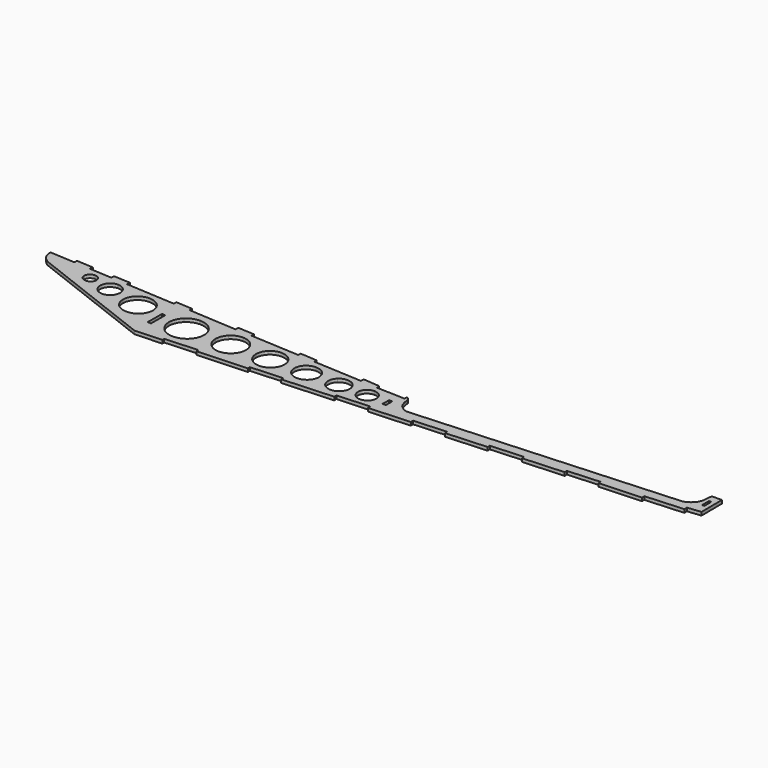
from build123d import *

# Parameters (mm, degrees)
F1_DEPTH = 3


# Not quite as in the source:
# - ends of sketch curves that miss each other by under 0.0002 mm in the source are joined
# - the dataset's text gives a spline's control points without its knots; the knots are read off the source's solid


with BuildPart() as f1:
    # F0 (on Top) → F1 (new body)
    with BuildSketch(Plane.XY):
        with BuildLine():
            Line((-283.705754, 26.242544), (-306.531989, 27.597216))
            Line((-306.531989, 27.597216), (-306.532132, 27.597217))
            add(Edge.make_bspline(
                [(-299.741399, 15.362947), (-303.248377, 18.203654), (-306.376642, 20.600294), (-306.532132, 27.597217)],
                knots=[0, 0, 0, 0, 1, 1, 1, 1], degree=3))
            Line((-299.741399, 15.362947), (-184.519619, -29.245478))
            Line((-184.519619, -29.245478), (-159.730079, -28.231688))
            Line((-159.730079, -28.231688), (-159.826994, -26.085226))
            Line((-159.826994, -26.085226), (-130.061797, -24.367861))
            Line((-130.061797, -24.367861), (-129.836804, -26.557253))
            Line((-129.836804, -26.557253), (-84.689902, -24.352981))
            Line((-84.689902, -24.352981), (-84.767699, -22.055153))
            Line((-84.767699, -22.055153), (-55.548697, -20.399041))
            Line((-55.548697, -20.399041), (-55.548607, -22.720141))
            Line((-55.548607, -22.720141), (-9.183299, -20.091946))
            Line((-9.183299, -20.091946), (-9.271814, -17.503366))
            Line((-9.271814, -17.503366), (20.343608, -15.913178))
            Line((20.343608, -15.913178), (20.340608, -18.583546))
            Line((20.340608, -18.583546), (57.798675, -16.459291))
            Line((57.798675, -16.459291), (57.7464, -13.835738))
            Line((57.7464, -13.835738), (87.580411, -12.096743))
            Line((87.580411, -12.096743), (87.59016, -14.588986))
            Line((87.59016, -14.588986), (124.670723, -12.419453))
            Line((124.670723, -12.419453), (124.718948, -9.896806))
            Line((124.718948, -9.896806), (154.696283, -8.076346))
            Line((154.696283, -8.076346), (154.845886, -10.628431))
            Line((154.845886, -10.628431), (191.943908, -8.450521))
            Line((191.943908, -8.450521), (191.926133, -5.905456))
            Line((191.926133, -5.905456), (221.443763, -4.073589))
            Line((221.443763, -4.073589), (221.435063, -6.558054))
            Line((221.435063, -6.558054), (259.473166, -4.558058))
            Line((259.473166, -4.558058), (259.447741, -1.913701))
            Line((259.447741, -1.913701), (294.319246, 0.265919))
            Line((294.319246, 0.265919), (294.223268, 3.278107))
            Line((294.223268, 3.278107), (306.532133, 4.590359))
            Line((306.532133, 4.590359), (306.343778, 28.117319))
            Line((306.343778, 28.117319), (298.342261, 27.997296))
            add(Edge.make_bspline(
                [(296.993228, 26.853134), (296.9935997444, 26.8539578555), (296.9936022923, 26.8539764219), (297.0233010775, 26.9195878034), (297.59233225, 28.1424128125), (298.342261, 27.997296)],
                knots=[0, 0, 0, 0, 0.0208333333, 0.03125, 1, 1, 1, 1], degree=3))
            Line((296.993228, 26.853134), (296.221861, 19.115617))
            add(Edge.make_bspline(
                [(285.733358, 8.770229), (290.415421, 10.119847), (295.053645, 13.441656), (296.221861, 19.115617)],
                knots=[0, 0, 0, 0, 1, 1, 1, 1], degree=3))
            Line((285.733358, 8.770229), (45.614513, -5.689073))
            add(Edge.make_bspline(
                [(38.011028, -1.579014), (40.407038, -3.364501), (42.648293, -5.614231), (45.614513, -5.689073)],
                knots=[0, 0, 0, 0, 1, 1, 1, 1], degree=3))
            add(Edge.make_bspline(
                [(34.690373, 8.210849), (35.274518, 4.947562), (35.678985, 1.684274), (38.011028, -1.579014)],
                knots=[0, 0, 0, 0, 1, 1, 1, 1], degree=3))
            add(Edge.make_bspline(
                [(31.92624, 11.727944), (33.14685, 10.854816), (34.877056, 10.491269), (34.690373, 8.210849)],
                knots=[0, 0, 0, 0, 1, 1, 1, 1], degree=3))
            Line((31.92624, 11.727944), (31.563826, 8.894204))
            Line((31.563826, 8.894204), (5.671996, 9.872969))
            Line((5.671996, 9.872969), (5.442765, 12.755872))
            Line((5.442765, 12.755872), (-9.382657, 14.013689))
            Line((-9.382657, 14.013689), (-9.615119, 10.891514))
            Line((-9.615119, 10.891514), (-53.849827, 13.259099))
            Line((-53.849827, 13.259099), (-54.080699, 15.881864))
            Line((-54.080699, 15.881864), (-69.487109, 16.950734))
            Line((-69.487109, 16.950734), (-69.592109, 14.198721))
            Line((-69.592109, 14.198721), (-114.174487, 16.652534))
            Line((-114.174487, 16.652534), (-114.050662, 19.463377))
            Line((-114.050662, 19.463377), (-129.098009, 20.234429))
            Line((-129.098009, 20.234429), (-129.237682, 17.136239))
            Line((-129.237682, 17.136239), (-173.38947, 19.880084))
            Line((-173.38947, 19.880084), (-173.40882, 22.677831))
            Line((-173.40882, 22.677831), (-188.406352, 23.557964))
            Line((-188.406352, 23.557964), (-188.417602, 20.663534))
            Line((-188.417602, 20.663534), (-233.27778, 23.322291))
            Line((-233.27778, 23.322291), (-233.11896, 26.423699))
            Line((-233.11896, 26.423699), (-248.233484, 27.111472))
            Line((-248.233484, 27.111472), (-248.199509, 24.138562))
            Line((-248.199509, 24.138562), (-268.624522, 25.372394))
            Line((-268.624522, 25.372394), (-268.486409, 28.327589))
            Line((-268.486409, 28.327589), (-283.648755, 29.245477))
            Line((-283.648755, 29.245477), (-283.705754, 26.242544))
        make_face()
        Polygon((-185.149065, -13.210493), (-184.989022, 2.952562), (-181.948447, 2.952562), (-181.948447, -13.370521), align=None, mode=Mode.SUBTRACT)
        with BuildLine():
            add(Edge.make_bspline(
                [(-157.220309, 11.895809), (-148.361018, 11.895807), (-141.179144, 4.900395), (-141.179144, -3.728881)],
                knots=[0, 0, 0, 0, 1, 1, 1, 1], degree=3))
            add(Edge.make_bspline(
                [(-141.179144, -3.728881), (-141.179142, -7.872807), (-142.869188, -11.847009), (-145.87749, -14.777209)],
                knots=[0, 0, 0, 0, 1, 1, 1, 1], degree=3))
            add(Edge.make_bspline(
                [(-145.87749, -14.777209), (-148.885792, -17.707408), (-152.965926, -19.353577), (-157.220309, -19.353578)],
                knots=[0, 0, 0, 0, 1, 1, 1, 1], degree=3))
            add(Edge.make_bspline(
                [(-157.220309, -19.353578), (-161.474694, -19.353579), (-165.55483, -17.707411), (-168.563134, -14.777211)],
                knots=[0, 0, 0, 0, 1, 1, 1, 1], degree=3))
            add(Edge.make_bspline(
                [(-168.563134, -14.777211), (-171.571438, -11.847012), (-173.261484, -7.872808), (-173.261482, -3.728881)],
                knots=[0, 0, 0, 0, 1, 1, 1, 1], degree=3))
            add(Edge.make_bspline(
                [(-173.261482, -3.728881), (-173.261482, 0.415045), (-171.571435, 4.389246), (-168.563131, 7.319444)],
                knots=[0, 0, 0, 0, 1, 1, 1, 1], degree=3))
            add(Edge.make_bspline(
                [(-168.563131, 7.319444), (-165.554828, 10.249642), (-161.474693, 11.89581), (-157.220309, 11.895809)],
                knots=[0, 0, 0, 0, 1, 1, 1, 1], degree=3))
        make_face(mode=Mode.SUBTRACT)
        with BuildLine():
            add(Edge.make_bspline(
                [(-107.474743, 6.629061), (-104.874921, 4.035491), (-103.414356, 0.517854), (-103.414357, -3.150008)],
                knots=[0, 0, 0, 0, 1, 1, 1, 1], degree=3))
            add(Edge.make_bspline(
                [(-103.414357, -3.150008), (-103.414359, -10.787934), (-109.621049, -16.979695), (-117.277387, -16.979694)],
                knots=[0, 0, 0, 0, 1, 1, 1, 1], degree=3))
            add(Edge.make_bspline(
                [(-117.277387, -16.979694), (-124.933725, -16.979695), (-131.140415, -10.787934), (-131.140417, -3.150008)],
                knots=[0, 0, 0, 0, 1, 1, 1, 1], degree=3))
            add(Edge.make_bspline(
                [(-131.140417, -3.150008), (-131.140418, 0.517854), (-129.679853, 4.035491), (-127.080031, 6.629061)],
                knots=[0, 0, 0, 0, 1, 1, 1, 1], degree=3))
            add(Edge.make_bspline(
                [(-127.080031, 6.629061), (-124.480208, 9.222632), (-120.954092, 10.679685), (-117.277387, 10.679684)],
                knots=[0, 0, 0, 0, 1, 1, 1, 1], degree=3))
            add(Edge.make_bspline(
                [(-117.277387, 10.679684), (-113.600682, 10.679685), (-110.074566, 9.222632), (-107.474743, 6.629061)],
                knots=[0, 0, 0, 0, 1, 1, 1, 1], degree=3))
        make_face(mode=Mode.SUBTRACT)
        with BuildLine():
            add(Edge.make_bspline(
                [(-71.752302, 5.620215), (-69.311057, 3.220874), (-67.939581, -0.033331), (-67.939582, -3.426511)],
                knots=[0, 0, 0, 0, 1, 1, 1, 1], degree=3))
            add(Edge.make_bspline(
                [(-67.939582, -3.426511), (-67.939585, -10.49244), (-73.767691, -16.220506), (-80.957025, -16.220506)],
                knots=[0, 0, 0, 0, 1, 1, 1, 1], degree=3))
            add(Edge.make_bspline(
                [(-80.957025, -16.220506), (-88.146358, -16.220506), (-93.974464, -10.49244), (-93.974467, -3.426511)],
                knots=[0, 0, 0, 0, 1, 1, 1, 1], degree=3))
            add(Edge.make_bspline(
                [(-93.974467, -3.426511), (-93.974468, -0.033331), (-92.602992, 3.220874), (-90.161747, 5.620215)],
                knots=[0, 0, 0, 0, 1, 1, 1, 1], degree=3))
            add(Edge.make_bspline(
                [(-90.161747, 5.620215), (-87.720503, 8.019556), (-84.409465, 9.367492), (-80.957025, 9.367492)],
                knots=[0, 0, 0, 0, 1, 1, 1, 1], degree=3))
            add(Edge.make_bspline(
                [(-80.957025, 9.367492), (-77.504584, 9.367492), (-74.193546, 8.019556), (-71.752302, 5.620215)],
                knots=[0, 0, 0, 0, 1, 1, 1, 1], degree=3))
        make_face(mode=Mode.SUBTRACT)
        with BuildLine():
            add(Edge.make_bspline(
                [(-11.024467, 3.097198), (-9.171185, 1.282396), (-8.130022, -1.179005), (-8.130022, -3.745524)],
                knots=[0, 0, 0, 0, 1, 1, 1, 1], degree=3))
            add(Edge.make_bspline(
                [(-8.130022, -3.745524), (-8.130022, -6.312042), (-9.171185, -8.773443), (-11.024467, -10.588245)],
                knots=[0, 0, 0, 0, 1, 1, 1, 1], degree=3))
            add(Edge.make_bspline(
                [(-11.024467, -10.588245), (-12.87775, -12.403048), (-15.39134, -13.422594), (-18.012277, -13.422594)],
                knots=[0, 0, 0, 0, 1, 1, 1, 1], degree=3))
            add(Edge.make_bspline(
                [(-18.012277, -13.422594), (-20.633214, -13.422594), (-23.146804, -12.403048), (-25.000087, -10.588245)],
                knots=[0, 0, 0, 0, 1, 1, 1, 1], degree=3))
            add(Edge.make_bspline(
                [(-25.000087, -10.588245), (-26.853369, -8.773443), (-27.894532, -6.312042), (-27.894532, -3.745524)],
                knots=[0, 0, 0, 0, 1, 1, 1, 1], degree=3))
            add(Edge.make_bspline(
                [(-27.894532, -3.745524), (-27.894532, -1.179005), (-26.853369, 1.282396), (-25.000087, 3.097198)],
                knots=[0, 0, 0, 0, 1, 1, 1, 1], degree=3))
            add(Edge.make_bspline(
                [(-25.000087, 3.097198), (-23.146804, 4.912001), (-20.633214, 5.931546), (-18.012277, 5.931546)],
                knots=[0, 0, 0, 0, 1, 1, 1, 1], degree=3))
            add(Edge.make_bspline(
                [(-18.012277, 5.931546), (-15.39134, 5.931546), (-12.87775, 4.912001), (-11.024467, 3.097198)],
                knots=[0, 0, 0, 0, 1, 1, 1, 1], degree=3))
        make_face(mode=Mode.SUBTRACT)
        with BuildLine():
            add(Edge.make_bspline(
                [(-39.874627, 4.160031), (-37.779004, 2.137357), (-36.601695, -0.605978), (-36.601695, -3.466471)],
                knots=[0, 0, 0, 0, 1, 1, 1, 1], degree=3))
            add(Edge.make_bspline(
                [(-36.601695, -3.466471), (-36.601695, -6.326964), (-37.779004, -9.070299), (-39.874627, -11.092973)],
                knots=[0, 0, 0, 0, 1, 1, 1, 1], degree=3))
            add(Edge.make_bspline(
                [(-39.874627, -11.092973), (-41.97025, -13.115648), (-44.812526, -14.251974), (-47.776185, -14.251974)],
                knots=[0, 0, 0, 0, 1, 1, 1, 1], degree=3))
            add(Edge.make_bspline(
                [(-47.776185, -14.251974), (-53.947682, -14.25197), (-58.950667, -9.423137), (-58.950667, -3.466471)],
                knots=[0, 0, 0, 0, 1, 1, 1, 1], degree=3))
            add(Edge.make_bspline(
                [(-58.950667, -3.466471), (-58.950667, 2.490195), (-53.947682, 7.319028), (-47.776185, 7.319032)],
                knots=[0, 0, 0, 0, 1, 1, 1, 1], degree=3))
            add(Edge.make_bspline(
                [(-47.776185, 7.319032), (-44.812526, 7.319032), (-41.97025, 6.182706), (-39.874627, 4.160031)],
                knots=[0, 0, 0, 0, 1, 1, 1, 1], degree=3))
        make_face(mode=Mode.SUBTRACT)
        with BuildLine():
            add(Edge.make_bspline(
                [(13.633606, 2.177433), (15.208477, 0.647132), (16.09323, -1.428402), (16.09323, -3.592576)],
                knots=[0, 0, 0, 0, 1, 1, 1, 1], degree=3))
            add(Edge.make_bspline(
                [(16.09323, -3.592576), (16.09323, -5.75675), (15.208477, -7.832284), (13.633606, -9.362585)],
                knots=[0, 0, 0, 0, 1, 1, 1, 1], degree=3))
            add(Edge.make_bspline(
                [(13.633606, -9.362585), (12.058734, -10.892887), (9.922751, -11.7526), (7.695548, -11.752599)],
                knots=[0, 0, 0, 0, 1, 1, 1, 1], degree=3))
            add(Edge.make_bspline(
                [(7.695548, -11.752599), (3.05764, -11.752598), (-0.702127, -8.099232), (-0.702127, -3.592576)],
                knots=[0, 0, 0, 0, 1, 1, 1, 1], degree=3))
            add(Edge.make_bspline(
                [(-0.702127, -3.592576), (-0.702127, 0.91408), (3.05764, 4.567446), (7.695548, 4.567447)],
                knots=[0, 0, 0, 0, 1, 1, 1, 1], degree=3))
            add(Edge.make_bspline(
                [(7.695548, 4.567447), (9.922751, 4.567448), (12.058734, 3.707735), (13.633606, 2.177433)],
                knots=[0, 0, 0, 0, 1, 1, 1, 1], degree=3))
        make_face(mode=Mode.SUBTRACT)
        Polygon((24.584311, -7.185893), (24.707168, 0.165757), (27.624871, 0.081726), (27.691171, -7.129343), align=None, mode=Mode.SUBTRACT)
        with BuildLine():
            add(Edge.make_bspline(
                [(-207.052605, 16.289564), (-199.516354, 16.289564), (-193.407016, 10.386583), (-193.407015, 3.104886)],
                knots=[0, 0, 0, 0, 1, 1, 1, 1], degree=3))
            add(Edge.make_bspline(
                [(-193.407015, 3.104886), (-193.407016, -4.17681), (-199.516354, -10.079791), (-207.052605, -10.079791)],
                knots=[0, 0, 0, 0, 1, 1, 1, 1], degree=3))
            add(Edge.make_bspline(
                [(-207.052605, -10.079791), (-214.588855, -10.079791), (-220.698193, -4.17681), (-220.698195, 3.104886)],
                knots=[0, 0, 0, 0, 1, 1, 1, 1], degree=3))
            add(Edge.make_bspline(
                [(-220.698195, 3.104886), (-220.698193, 10.386583), (-214.588855, 16.289564), (-207.052605, 16.289564)],
                knots=[0, 0, 0, 0, 1, 1, 1, 1], degree=3))
        make_face(mode=Mode.SUBTRACT)
        with BuildLine():
            add(Edge.make_bspline(
                [(-237.755804, 18.777554), (-232.739156, 18.777554), (-228.672359, 14.71945), (-228.672359, 9.713527)],
                knots=[0, 0, 0, 0, 1, 1, 1, 1], degree=3))
            add(Edge.make_bspline(
                [(-228.672359, 9.713527), (-228.672359, 4.707603), (-232.739156, 0.649499), (-237.755804, 0.649499)],
                knots=[0, 0, 0, 0, 1, 1, 1, 1], degree=3))
            add(Edge.make_bspline(
                [(-237.755804, 0.649499), (-240.164885, 0.649497), (-242.475297, 1.604454), (-244.178775, 3.304289)],
                knots=[0, 0, 0, 0, 1, 1, 1, 1], degree=3))
            add(Edge.make_bspline(
                [(-244.178775, 3.304289), (-245.882253, 5.004124), (-246.839257, 7.309596), (-246.839257, 9.713527)],
                knots=[0, 0, 0, 0, 1, 1, 1, 1], degree=3))
            add(Edge.make_bspline(
                [(-246.839257, 9.713527), (-246.839257, 12.117457), (-245.882253, 14.422929), (-244.178775, 16.122764)],
                knots=[0, 0, 0, 0, 1, 1, 1, 1], degree=3))
            add(Edge.make_bspline(
                [(-244.178775, 16.122764), (-242.475297, 17.822599), (-240.164885, 18.777556), (-237.755804, 18.777554)],
                knots=[0, 0, 0, 0, 1, 1, 1, 1], degree=3))
        make_face(mode=Mode.SUBTRACT)
        with BuildLine():
            add(Edge.make_bspline(
                [(-259.619677, 19.814587), (-256.513777, 19.814588), (-253.995946, 17.423667), (-253.995945, 14.474317)],
                knots=[0, 0, 0, 0, 1, 1, 1, 1], degree=3))
            add(Edge.make_bspline(
                [(-253.995945, 14.474317), (-253.995946, 11.524966), (-256.513777, 9.134045), (-259.619677, 9.134047)],
                knots=[0, 0, 0, 0, 1, 1, 1, 1], degree=3))
            add(Edge.make_bspline(
                [(-259.619677, 9.134047), (-262.725577, 9.134045), (-265.243408, 11.524966), (-265.24341, 14.474317)],
                knots=[0, 0, 0, 0, 1, 1, 1, 1], degree=3))
            add(Edge.make_bspline(
                [(-265.24341, 14.474317), (-265.243408, 17.423667), (-262.725577, 19.814588), (-259.619677, 19.814587)],
                knots=[0, 0, 0, 0, 1, 1, 1, 1], degree=3))
        make_face(mode=Mode.SUBTRACT)
        Polygon((300.222668, 13.034459), (300.222653, 21.035976), (302.303056, 20.995927), (302.303056, 13.074434), align=None, mode=Mode.SUBTRACT)
    extrude(amount=F1_DEPTH)


solid = f1.part
